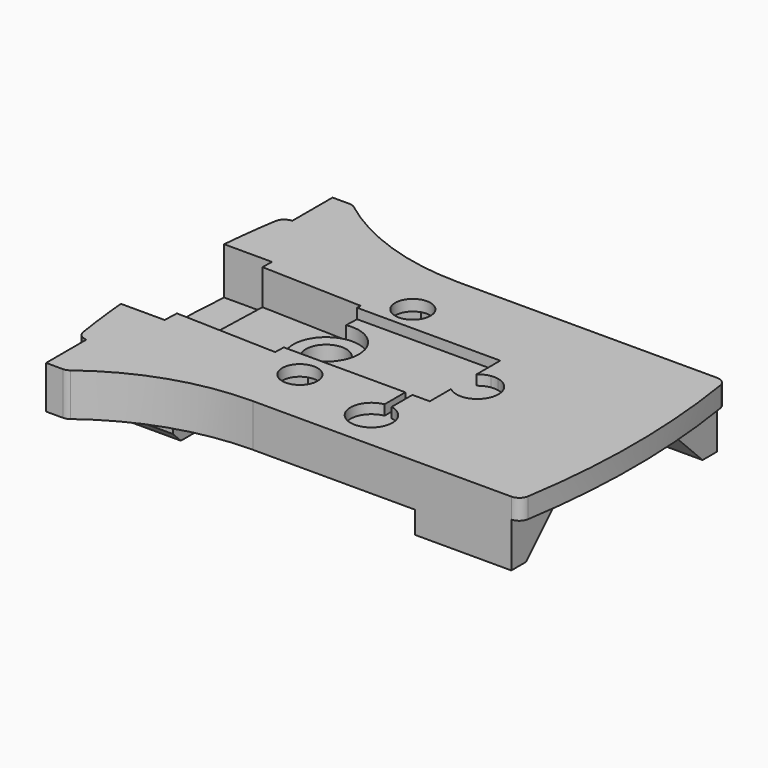
from build123d import *

# Parameters (mm, degrees)
F1_DEPTH     = 2
F2_R         = 1
F4_DEPTH     = 2.25
F6_DEPTH     = 2.2
F7_R         = 2
F8_DEPTH     = 25
F9_R         = 3.25
F9_R_2       = 2
F10_DEPTH    = 2.25
F12_DEPTH    = 4.65
F14_DEPTH    = 3.5
F16_DEPTH    = 1
F17_R        = 1.75
F18_DEPTH    = 25
F20_DEPTH    = 3.15
F21_W        = 9.561190108
F21_H        = 6.25
F22_DEPTH    = 4.45
F23_T4_DEPTH = 21.0051794045
F23_T9_DEPTH = 21.0051794045
F24_SIZE     = 1
F26_DEPTH    = 4.25
F27_R        = 1


# Not quite as in the source:
# - a fillet or chamfer that OpenCascade refuses, or shapes differently, is made with other operations: its cross-section is extruded or revolved along the edge and cut away or added
# - a pattern or mirror of a feature is missing from the dataset's text; its kind, count and spacing are read off the source's solid


with BuildPart() as f1:
    # F0 (on Top) → F1 (new body)
    with BuildSketch(Plane.XY):
        with BuildLine():
            Line((21.9083046755, 12.75), (-21.9083046755, 12.75))
            ThreePointArc((-21.9083046755, 12.75), (-23, 0), (-21.9083046755, -12.75))
            Line((-21.9083046755, -12.75), (21.9083046755, -12.75))
            ThreePointArc((21.9083046755, -12.75), (23, 0), (21.9083046755, 12.75))
        make_face()
    extrude(amount=F1_DEPTH)

    # F2
    f2_edges = [f1.edges().sort_by_distance(p)[0] for p in [
        (-21.908305, 12.75, 1),
        (21.908305, 12.75, 1),
        (-21.908305, -12.75, 1),
        (21.908305, -12.75, 1),
    ]]
    fillet(f2_edges, radius=F2_R)

    # F3 (on face) → F4 (join)
    with BuildSketch(Plane(origin=(0, 0, 0), x_dir=(1, 0, 0), z_dir=(0, 0, -1))):
        with BuildLine():
            Line((11.5, 12.75), (-21.061190108, 12.75))
            ThreePointArc((-21.061190108, 12.75), (-21.7097331737, 12.5111779634), (-22.0485034879, 11.9087837838))
            ThreePointArc((-22.0485034879, 11.9087837838), (-23, 0), (-22.0485034879, -11.9087837838))
            ThreePointArc((-22.0485034879, -11.9087837838), (-21.7097331737, -12.5111779634), (-21.061190108, -12.75))
            Line((-21.061190108, -12.75), (11.5, -12.75))
            Line((11.5, -12.75), (11.5, 12.75))
        make_face()
    extrude(amount=F4_DEPTH)

    # F5 (on face) → F6 (join)
    with BuildSketch(Plane(origin=(0, 0, -2.25), x_dir=(1, 0, 0), z_dir=(0, 0, -1))):
        with BuildLine():
            ThreePointArc((-22.0485034879, -11.9087837838), (-21.7097331737, -12.5111779634), (-21.061190108, -12.75))
            Line((-21.061190108, -12.75), (-12.5, -12.75))
            Line((-12.5, -12.75), (-12.5, 12.75))
            Line((-12.5, 12.75), (-21.061190108, 12.75))
            ThreePointArc((-21.061190108, 12.75), (-21.7097331737, 12.5111779634), (-22.0485034879, 11.9087837838))
            ThreePointArc((-22.0485034879, 11.9087837838), (-23, 0), (-22.0485034879, -11.9087837838))
        make_face()
    extrude(amount=F6_DEPTH)

    # F7 (on face) → F8 (cut)
    with BuildSketch(Plane(origin=(0, 0, -2.25), x_dir=(1, 0, 0), z_dir=(0, 0, -1))):
        with Locations((-7.5, 0)):
            Circle(F7_R)
    extrude(amount=-F8_DEPTH, mode=Mode.SUBTRACT)

    # F9 (on face) → F10 (cut)
    with BuildSketch(Plane.XY.offset(2)):
        with Locations((-7.5, 0)):
            Circle(F9_R)
        with Locations((-7.5, 0)):
            Circle(F9_R_2, mode=Mode.SUBTRACT)
    extrude(amount=-F10_DEPTH, mode=Mode.SUBTRACT)

    # F11 (on face) → F12 (cut)
    with BuildSketch(Plane.XY.offset(2)):
        Polygon((-17.9767161827, 6.3967091968), (-22.7267161827, 6.3967091968), (-22.7267161827, -6.3967091968), (-18.3871376794, -6.3967091968), align=None)
        with BuildLine():
            ThreePointArc((-22.7267161827, -6.3967091968), (-23, 0), (-22.7267161827, 6.3967091968))
            Line((-22.7267161827, 6.3967091968), (-24.9030976, 6.3967091968))
            Line((-24.9030976, 6.3967091968), (-24.9030976, -6.3967091968))
            Line((-24.9030976, -6.3967091968), (-23.1371376794, -6.3967091968))
            Line((-23.1371376794, -6.3967091968), (-22.7267161827, -6.3967091968))
        make_face()
        Polygon((-22.7267161827, -6.3967091968), (-22.7267161827, 6.3967091968), (-24.9030976, 6.3967091968), (-24.9030976, -6.3967091968), (-23.1371376794, -6.3967091968), align=None)
    extrude(amount=-F12_DEPTH, mode=Mode.SUBTRACT)

    # F13 (on face) → F14 (cut)
    with BuildSketch(Plane.XY.offset(2)):
        with BuildLine():
            Line((-8.0183982933, 4.9370567441), (-18.0132564134, 5.2576985384))
            Line((-18.0132564134, 5.2576985384), (-18.3403110436, -4.9370567441))
            Line((-18.3403110436, -4.9370567441), (-8.3454529235, -5.2576985384))
            Line((-8.3454529235, -5.2576985384), (-8.2780130541, -3.1555024462))
            ThreePointArc((-8.2780130541, -3.1555024462), (-10.748328889, 0.1042085831), (-8.074160142, 3.1988810749))
            Line((-8.074160142, 3.1988810749), (-8.0183982933, 4.9370567441))
        make_face()
    extrude(amount=-F14_DEPTH, mode=Mode.SUBTRACT)

    # F15 (on face) → F16 (cut)
    with BuildSketch(Plane.XY.offset(2)):
        with BuildLine():
            ThreePointArc((7.2010516835, -2.053352114), (7.5517942695, -2.0743534785), (7.9010516835, -2.0358739026))
            ThreePointArc((7.9010516835, -2.0358739026), (9.575, 0), (7.9010516835, 2.0358739026))
            ThreePointArc((7.9010516835, 2.0358739026), (7.5517942695, 2.0743534785), (7.2010516835, 2.053352114))
            ThreePointArc((7.2010516835, 2.053352114), (6.646380727, 1.8912850491), (6.1579127796, 1.5825381173))
            Line((6.1579127796, 1.5825381173), (6.1579127796, 4.5080841794))
            Line((6.1579127796, 4.5080841794), (-8.312298453, 4.5080841794))
            Line((-8.312298453, 4.5080841794), (-8.312298453, -4.22422681))
            Line((-8.312298453, -4.22422681), (3.735084728, -4.22422681))
            Line((3.735084728, -4.22422681), (3.735084728, -6.8032004514))
            ThreePointArc((3.735084728, -6.8032004514), (4.0668227554, -10.9249796186), (4.435084728, -6.8063030421))
            Line((4.435084728, -6.8063030421), (4.435084728, -4.22422681))
            Line((4.435084728, -4.22422681), (6.1579127796, -4.22422681))
            Line((6.1579127796, -4.22422681), (6.1579127796, -1.5825381173))
            ThreePointArc((6.1579127796, -1.5825381173), (6.646380727, -1.8912850491), (7.2010516835, -2.053352114))
        make_face()
    extrude(amount=-F16_DEPTH, mode=Mode.SUBTRACT)

    # F17 (on face) → F18 (cut)
    with BuildSketch(Plane.XY.offset(2)):
        with Locations((-4.5, 7)):
            Circle(F17_R)
        with Locations((-4.5, -7)):
            Circle(F17_R)
    extrude(amount=-F18_DEPTH, mode=Mode.SUBTRACT)

    # F19 (on face) → F20 (cut)
    with BuildSketch(Plane(origin=(0, 0, -2.25), x_dir=(1, 0, 0), z_dir=(0, 0, -1))):
        Polygon((-2.4359727876, 10.575), (-6.5640272124, 10.575), (-8.6280544247, 7), (-6.5640272124, 3.425), (-2.4359727876, 3.425), (-0.3719455753, 7), align=None)
        Polygon((-2.4359727876, -3.425), (-6.5640272124, -3.425), (-8.6280544247, -7), (-6.5640272124, -10.575), (-2.4359727876, -10.575), (-0.3719455753, -7), align=None)
    extrude(amount=-F20_DEPTH, mode=Mode.SUBTRACT)

    # F21 (on face) → F22 (join, through all)
    with BuildSketch(Plane(origin=(0, 0, 0), x_dir=(1, 0, 0), z_dir=(0, 0, -1))):
        with Locations((16.280595054, 9.625)):
            Rectangle(F21_W, F21_H)
        with Locations((16.280595054, -9.625)):
            Rectangle(F21_W, F21_H)
    extrude(amount=F22_DEPTH)

    # F23: chamfer of 4.45 on 2 edges, made by hand


with BuildPart() as f23_tool2:
    # F23_s3 → F23_t4 (new body)
    with BuildSketch(Plane.YZ.offset(11.5)):
        Polygon((-6.5, 0), (-10.95, -4.45), (-6.5, -4.45), align=None)
    extrude(amount=F23_T4_DEPTH)

    split(bisect_by=Plane.XY, keep=Keep.BOTTOM)


with BuildPart() as f1_1:
    add(f1.part)

    # F23_t1: cut F23_tool2
    add(f23_tool2.part, mode=Mode.SUBTRACT)


with BuildPart() as f23_tool7:
    # F23_s8 → F23_t9 (new body)
    with BuildSketch(Plane.YZ.offset(32.5051794045)):
        Polygon((10.95, -4.45), (6.5, 0), (6.5, -4.45), align=None)
    extrude(amount=-F23_T9_DEPTH)

    split(bisect_by=Plane.XY, keep=Keep.BOTTOM)


with BuildPart() as f1_2:
    add(f1_1.part)

    # F23_t6: cut F23_tool7
    add(f23_tool7.part, mode=Mode.SUBTRACT)

    # F24
    f24_edges = [f1_2.edges().sort_by_distance(p)[0] for p in [
        (-16.780595, -12.75, -4.45),
        (-16.780595, 12.75, -4.45),
        (-21.709733, -12.511178, -4.45),
        (-23, 0, -4.45),
        (-21.709733, 12.511178, -4.45),
    ]]
    chamfer(f24_edges, length=F24_SIZE)

    # F25 (on face) → F26 (join, through all)
    with BuildSketch(Plane.XY.offset(2)):
        with BuildLine():
            Line((-21.061190108, 17.75), (-21.061190108, 12.75))
            Line((-21.061190108, 12.75), (-4.561190108, 12.75))
            ThreePointArc((-4.561190108, 12.75), (-12.2301209331, 14.0351006072), (-19.061190108, 17.75))
            Line((-19.061190108, 17.75), (-21.061190108, 17.75))
        make_face()
    f26 = extrude(amount=-F26_DEPTH)

    # F26_copies: F26 across plane
    add(f26.mirror(Plane(origin=(0, 0, 0), x_dir=(0, 0, -1), z_dir=(0, -1, 0))))

    # F27
    f27_edges = [f1_2.edges().sort_by_distance(p)[0] for p in [
        (-19.06119, 17.75, -0.125),
        (-19.06119, -17.75, -0.125),
    ]]
    fillet(f27_edges, radius=F27_R)


solid = f1_2.part
